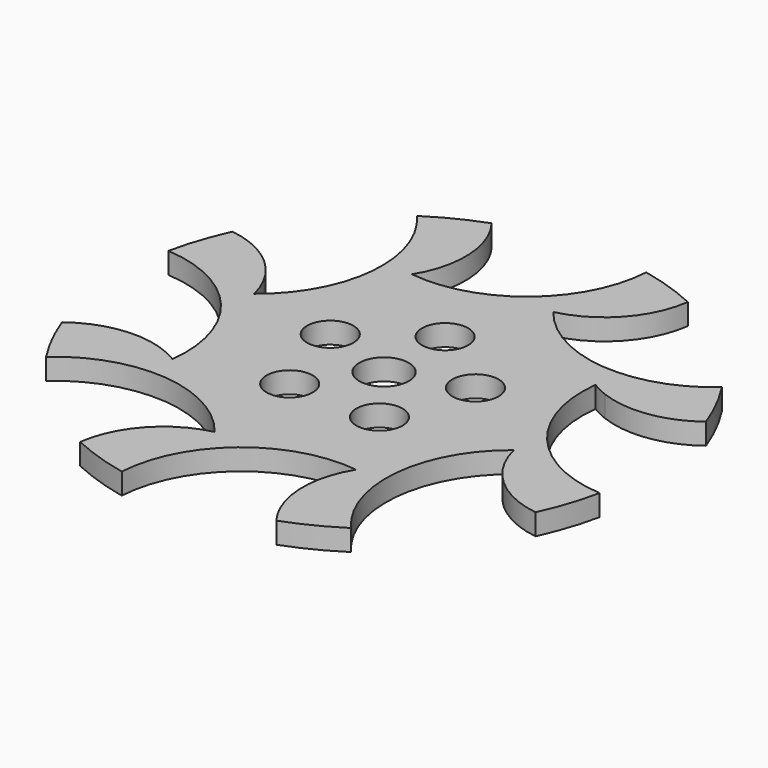
from build123d import *

# Parameters (mm, degrees)
F0_R     = 3.2677789254
F0_R_2   = 3.5
F1_DEPTH = 3


# Not quite as in the source:
# - a feature names something its author has since deleted; it is built from what else it names


with BuildPart() as f1:
    # F0 (on Top) → F1 (new body)
    with BuildSketch(Plane.XY):
        with BuildLine():
            ThreePointArc((-12.185161002, 20.1667081565), (-10.2249151213, 27.7991061308), (-12.9275786797, 35.2012458513))
            ThreePointArc((-12.9275786797, 35.2012458513), (-16.80912748, 33.5216830329), (-20.4768659437, 31.4157279261))
            ThreePointArc((-20.4768659437, 31.4157279261), (-16.1164151017, 18.0121200855), (-22.876226066, 5.6438061173))
            ThreePointArc((-22.876226066, 5.6438061173), (-26.8870432753, 12.4268296367), (-34.0322181964, 15.7498610989))
            ThreePointArc((-34.0322181964, 15.7498610989), (-35.5892574163, 11.8175613624), (-36.6936050187, 7.7349434862))
            ThreePointArc((-36.6936050187, 7.7349434862), (-24.1325186628, 1.3404658492), (-20.1667081565, -12.185161002))
            ThreePointArc((-20.1667081565, -12.185161002), (-27.7991061308, -10.2249151213), (-35.2012458513, -12.9275786797))
            ThreePointArc((-35.2012458513, -12.9275786797), (-33.5216830329, -16.80912748), (-31.4157279261, -20.4768659437))
            ThreePointArc((-31.4157279261, -20.4768659437), (-18.0121200855, -16.1164151017), (-5.6438061173, -22.876226066))
            ThreePointArc((-5.6438061173, -22.876226066), (-12.4268296367, -26.8870432753), (-15.7498610989, -34.0322181964))
            ThreePointArc((-15.7498610989, -34.0322181964), (-11.8175613624, -35.5892574163), (-7.7349434862, -36.6936050187))
            ThreePointArc((-7.7349434862, -36.6936050187), (-1.3404658492, -24.1325186628), (12.185161002, -20.1667081565))
            ThreePointArc((12.185161002, -20.1667081565), (10.2249151213, -27.7991061308), (12.9275786797, -35.2012458513))
            ThreePointArc((12.9275786797, -35.2012458513), (16.80912748, -33.5216830329), (20.4768659437, -31.4157279261))
            ThreePointArc((20.4768659437, -31.4157279261), (16.1164151017, -18.0121200855), (22.876226066, -5.6438061173))
            ThreePointArc((22.876226066, -5.6438061173), (26.8870432753, -12.4268296367), (34.0322181964, -15.7498610989))
            ThreePointArc((34.0322181964, -15.7498610989), (35.5892574163, -11.8175613624), (36.6936050187, -7.7349434862))
            ThreePointArc((36.6936050187, -7.7349434862), (24.1325186628, -1.3404658492), (20.1667081565, 12.185161002))
            ThreePointArc((20.1667081565, 12.185161002), (21.2681317348, 11.5765458519), (22.4221424931, 11.0747436302))
            ThreePointArc((22.4221424931, 11.0747436302), (29.051621985, 10.3463660778), (35.2012458513, 12.9275786797))
            ThreePointArc((35.2012458513, 12.9275786797), (33.5216830329, 16.80912748), (31.4157279261, 20.4768659437))
            ThreePointArc((31.4157279261, 20.4768659437), (18.0121200855, 16.1164151017), (5.6438061173, 22.876226066))
            ThreePointArc((5.6438061173, 22.876226066), (12.4268296367, 26.8870432753), (15.7498610989, 34.0322181964))
            ThreePointArc((15.7498610989, 34.0322181964), (11.8175613624, 35.5892574163), (7.7349434862, 36.6936050187))
            ThreePointArc((7.7349434862, 36.6936050187), (1.3404658492, 24.1325186628), (-12.185161002, 20.1667081565))
        make_face()
        with Locations((-6.3489950769, -8.7386420371)):
            Circle(F0_R, mode=Mode.SUBTRACT)
        with Locations((6.3489950769, -8.7386420371)):
            Circle(F0_R, mode=Mode.SUBTRACT)
        with Locations((-10.2728898289, 3.3378642426)):
            Circle(F0_R, mode=Mode.SUBTRACT)
        Circle(F0_R_2, mode=Mode.SUBTRACT)
        with Locations((10.2728898289, 3.3378642426)):
            Circle(F0_R, mode=Mode.SUBTRACT)
        with Locations((0, 10.8015555888)):
            Circle(F0_R, mode=Mode.SUBTRACT)
    extrude(amount=F1_DEPTH)


solid = f1.part
